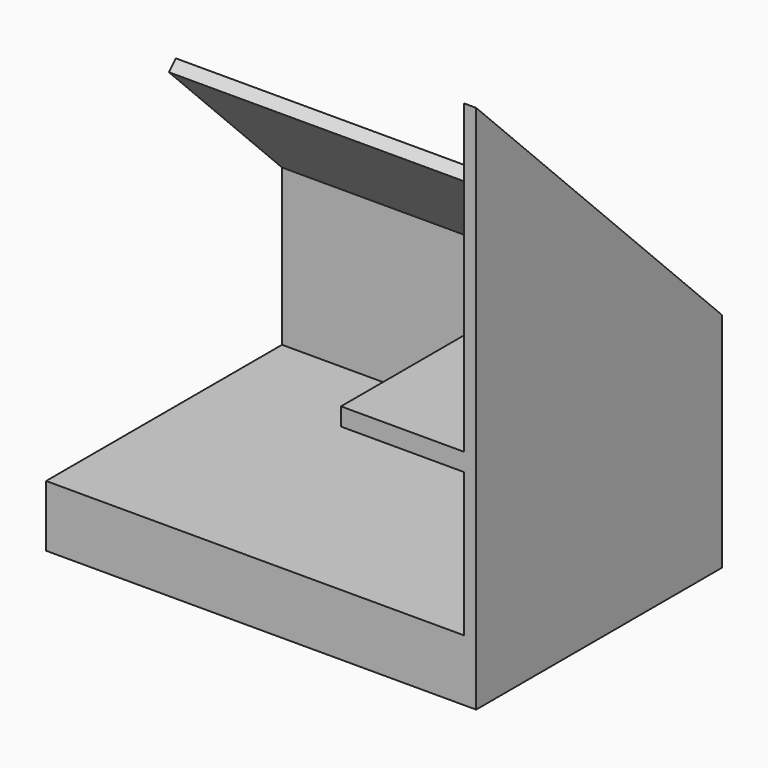
from build123d import *

# Parameters (mm, degrees)
F0_W      = 7000
F0_H      = 5000
F1_DEPTH  = 1000
F3_DEPTH  = 2300
F5_DEPTH  = 6800
F6_REACH  = 7685.420757516
F7_W      = 2580
F7_H      = 290
F8_DEPTH  = 2000
F10_DEPTH = 700
F12_DEPTH = 700
F13_W     = 800
F13_H     = 1100
F14_DEPTH = 200.001
F15_W     = 100
F15_H     = 100
F16_DEPTH = 2200
F18_START = 25
F18_DEPTH = 50
F19_W     = 100
F19_H     = 100
F20_DEPTH = 1236
F23_DEPTH = 50
F25_DEPTH = 50
F26_START = 25
F26_DEPTH = 50
F27_R     = 20
F27_2_R   = 20


with BuildPart() as f1:
    # F0 (on Top) → F1 (new body)
    with BuildSketch(Plane.XY):
        Rectangle(F0_W, F0_H)
    extrude(amount=-F1_DEPTH)

    # F2 (on face) → F3 (join)
    with BuildSketch(Plane.XY):
        Polygon((3500, -2500), (3500, 2500), (-3500, 2500), (-3500, 2300), (3300, 2300), (3300, -2500), align=None)
    extrude(amount=F3_DEPTH)

    # F4 (on face) → F5 (join, through all)
    with BuildSketch(Plane(origin=(3300, 0, 0), x_dir=(0, -1, 0), z_dir=(-1, 0, 0))):
        Polygon((-2300, 2300), (-2300, 2540), (0, 4840), (-141.4213562373, 4981.4213562373), (-2500, 2622.8427124746), (-2500, 2300), align=None)
    extrude(amount=F5_DEPTH)

    f6_end = Plane(origin=(-100, 1320.7106781187, 3802.132034356), x_dir=(0, -0.7071067812, 0.7071067812), z_dir=(0, 0.7071067812, 0.7071067812))
    # F3_face (on face) → F6 (join, up to a plane its end follows)
    with BuildSketch(Plane(origin=(3400, 0, 2300), x_dir=(1, 0, 0), z_dir=(0, 0, 1))):
        Polygon((-100, -2500), (100, -2500), (100, 2500), (-100, 2500), (-100, 2300), align=None)
    f6_long = extrude(amount=F6_REACH, mode=Mode.PRIVATE)
    add(split(f6_long, bisect_by=f6_end, keep=Keep.BOTTOM, mode=Mode.PRIVATE))

    # F7 (on face) → F8 (join)
    with BuildSketch(Plane(origin=(3300, 0, 0), x_dir=(0, -1, 0), z_dir=(-1, 0, 0))):
        with Locations((1210, 2485)):
            Rectangle(F7_W, F7_H)
    extrude(amount=F8_DEPTH)

    # F13 (on face) → F14 (cut, through all)
    with BuildSketch(Plane.XZ.offset(-2300)):
        with Locations((2430, 1475)):
            Rectangle(F13_W, F13_H)
    extrude(amount=-F14_DEPTH, mode=Mode.SUBTRACT)


with BuildPart() as f10:
    # F9 (on face) → F10 (new body)
    with BuildSketch(Plane(origin=(3300, 0, 0), x_dir=(0, -1, 0), z_dir=(-1, 0, 0))):
        Polygon((-80, 2427.7), (-290, 2427.7), (-290, 2225.4), (-500, 2225.4), (-500, 2023.1), (-710, 2023.1), (-710, 1820.8), (-920, 1820.8), (-920, 1618.5), (-1130, 1618.5), (-1130, 1416.2), (-1340, 1416.2), (-1340, 1213.9), (-1550, 1213.9), (-1550, 1011.6), (-2300, 1011.6), (-2300, 911.6), (-1550, 911.6), (-1550, 936.1943204678), (-80, 2352.2943204678), align=None)
    extrude(amount=F10_DEPTH)


with BuildPart() as f12:
    # F11 (on face) → F12 (new body)
    with BuildSketch(Plane.XZ.offset(-2300)):
        Polygon((2600, 733.8943204678), (2600, 809.3), (2390, 809.3), (2390, 607), (2180, 607), (2180, 404.7), (1970, 404.7), (1970, 202.4), (1760, 202.4), (1760, 0.1), (1550, 0.1), (1550, -202.2), (1838.1719856736, 0), align=None)
    extrude(amount=F12_DEPTH)


with BuildPart() as f16:
    # F15 (on face) → F16 (new body)
    with BuildSketch(Plane.XY):
        with Locations((2550, 1550)):
            Rectangle(F15_W, F15_H)
    extrude(amount=F16_DEPTH)

    # F17 (on face) → F18 (join)
    with BuildSketch(Plane(origin=(2600, 0, 0), x_dir=(0, -1, 0), z_dir=(-1, 0, 0)).offset(F18_START)):
        Polygon((-80, 3530), (-1500, 2162.0666666667), (-1500, 2050.9843948538), (-80, 3418.9177281871), align=None)
    extrude(amount=F18_DEPTH)

    # F27
    f27_edges = [f16.edges().sort_by_distance(p)[0] for p in [
        (2525, 790, 2846.033333),
        (2575, 790, 2846.033333),
    ]]
    fillet(f27_edges, radius=F27_R)


with BuildPart() as f20:
    # F19 (on face) → F20 (new body)
    with BuildSketch(Plane(origin=(0, 0, 0), x_dir=(1, 0, 0), z_dir=(0, 0, -1))):
        with Locations((1810, -1550)):
            Rectangle(F19_W, F19_H)
    extrude(amount=-F20_DEPTH)


with BuildPart() as f23:
    # F22 (on face) → F23 (new body)
    with BuildSketch(Plane.XZ.offset(-1600)):
        Polygon((2390, 607), (2390, 809.3), (2180, 607), align=None)
        Polygon((1860, 202.4), (1860, 21.0276538011), (2500, 637.5609871345), (2500, 809.3), (2390, 809.3), (2390, 607), (2180, 607), (2180, 404.7), (1970, 404.7), (1970, 202.4), align=None)
        Polygon((2180, 607), (1970, 404.7), (2180, 404.7), align=None)
        Polygon((1860, 298.7333333333), (1860, 202.4), (1970, 202.4), (1970, 404.7), align=None)
        Polygon((2390, 809.3), (2500, 809.3), (2500, 915.2666666667), align=None)
    extrude(amount=F23_DEPTH)


with BuildPart() as f25:
    # F24 (on face) → F25 (new body)
    with BuildSketch(Plane(origin=(2600, 0, 0), x_dir=(0, -1, 0), z_dir=(-1, 0, 0))):
        Polygon((-1500, 1262.0666666667), (-1500, 984.3609871345), (-80, 2352.2943204678), (-80, 2630), align=None)
    extrude(amount=F25_DEPTH)


with BuildPart() as f26:
    # F21 (on face) → F26 (new body)
    with BuildSketch(Plane.XZ.offset(-1600).offset(F26_START)):
        Polygon((2500, 1815.2666666667), (1860, 1198.7333333333), (1860, 1087.6510615204), (2500, 1704.1843948538), align=None)
    extrude(amount=F26_DEPTH)

    # F27#2
    f27_2_edges = [f26.edges().sort_by_distance(p)[0] for p in [
        (2180, 1575, 1507),
        (2180, 1525, 1507),
    ]]
    fillet(f27_2_edges, radius=F27_2_R)


solid = Compound([f1.part, f10.part, f12.part, f16.part, f20.part, f23.part, f25.part, f26.part])
